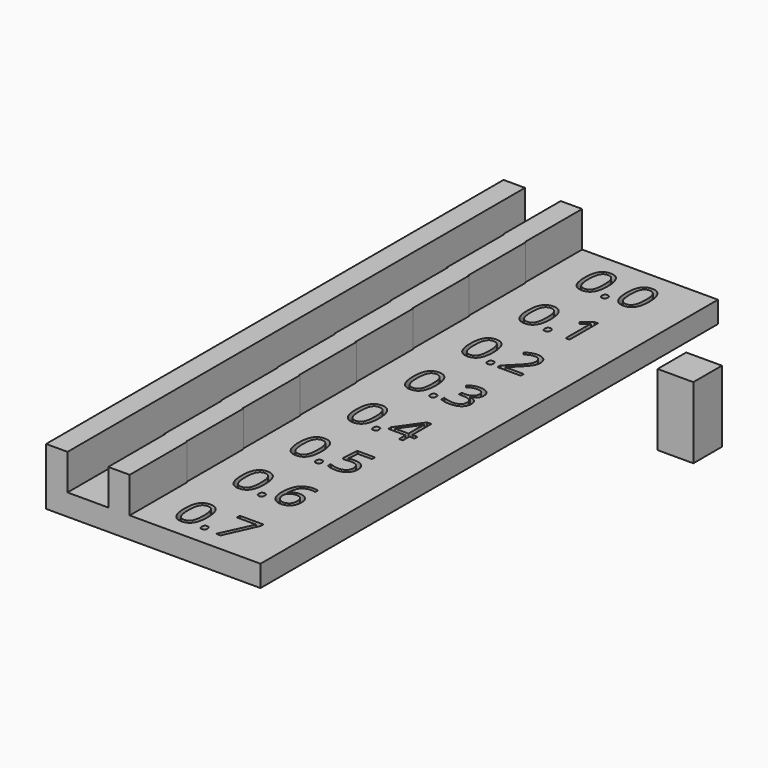
from build123d import *

# Parameters (mm, degrees)
F0_W         = 30
F0_H         = 80
F1_DEPTH     = 3
F2_W         = 3
F2_H         = 80
F3_DEPTH     = 5
F4_TEXT_SIZE = 6.9444444444
F5_DEPTH     = 1
F6_W         = 5
F6_H         = 5
F7_DEPTH     = 10


# Not quite as in the source:
# - Text() gives the source's letters only with a copy of the font that has no kerning and outlines rounded to 1/6400 em; it was checked with that copy


with BuildPart() as f1:
    # F0 (on Top) → F1 (new body)
    with BuildSketch(Plane.XY):
        Rectangle(F0_W, F0_H)
    extrude(amount=F1_DEPTH)

    # F2 (on face) → F3 (join)
    with BuildSketch(Plane.XY.offset(3)):
        Polygon((-4, 40), (-7, 40), (-7, 30), (-6.9, 30), (-4, 30), align=None)
        Polygon((-4, 30), (-6.9, 30), (-6.9, 20), (-6.8, 20), (-3.9, 20), (-3.9, 30), align=None)
        Polygon((-3.9, 20), (-6.8, 20), (-6.8, 10), (-6.7, 10), (-3.8, 10), (-3.8, 20), align=None)
        Polygon((-3.8, 10), (-6.7, 10), (-6.7, 0), (-6.6, 0), (-3.7, 0), (-3.7, 10), align=None)
        Polygon((-6.6, -10), (-6.5, -10), (-3.6, -10), (-3.6, 0), (-3.7, 0), (-6.6, 0), align=None)
        Polygon((-6.5, -20), (-6.4, -20), (-3.5, -20), (-3.5, -10), (-3.6, -10), (-6.5, -10), align=None)
        Polygon((-6.4, -30), (-6.3, -30), (-3.4, -30), (-3.4, -20), (-3.5, -20), (-6.4, -20), align=None)
        Polygon((-6.3, -30), (-6.3, -40), (-3.3, -40), (-3.3, -30), (-3.4, -30), align=None)
        with Locations((-13.5, 0)):
            Rectangle(F2_W, F2_H)
    extrude(amount=F3_DEPTH)

    # F4 (on face) → F5 (cut)
    with BuildSketch(Plane.XY.offset(3)):
        with Locations((0, 32.5)):
            Text('0.0', F4_TEXT_SIZE, font='Open Sans', text_align=(TextAlign.LEFT, TextAlign.BOTTOM))
        with Locations((0, 22.5)):
            Text('0.1', F4_TEXT_SIZE, font='Open Sans', text_align=(TextAlign.LEFT, TextAlign.BOTTOM))
        with Locations((0, 12.5)):
            Text('0.2', F4_TEXT_SIZE, font='Open Sans', text_align=(TextAlign.LEFT, TextAlign.BOTTOM))
        with Locations((0, 2.5)):
            Text('0.3', F4_TEXT_SIZE, font='Open Sans', text_align=(TextAlign.LEFT, TextAlign.BOTTOM))
        with Locations((0, -7.5)):
            Text('0.4', F4_TEXT_SIZE, font='Open Sans', text_align=(TextAlign.LEFT, TextAlign.BOTTOM))
        with Locations((0, -17.5)):
            Text('0.5', F4_TEXT_SIZE, font='Open Sans', text_align=(TextAlign.LEFT, TextAlign.BOTTOM))
        with Locations((0, -27.5)):
            Text('0.6', F4_TEXT_SIZE, font='Open Sans', text_align=(TextAlign.LEFT, TextAlign.BOTTOM))
        with Locations((0, -37.5)):
            Text('0.7', F4_TEXT_SIZE, font='Open Sans', text_align=(TextAlign.LEFT, TextAlign.BOTTOM))
    extrude(amount=-F5_DEPTH, mode=Mode.SUBTRACT)


with BuildPart() as f7:
    # F6 (on Top) → F7 (new body)
    with BuildSketch(Plane.XY):
        with Locations((30.9821417928, 15.0892860815)):
            Rectangle(F6_W, F6_H)
    extrude(amount=F7_DEPTH)


solid = Compound([f1.part, f7.part])
